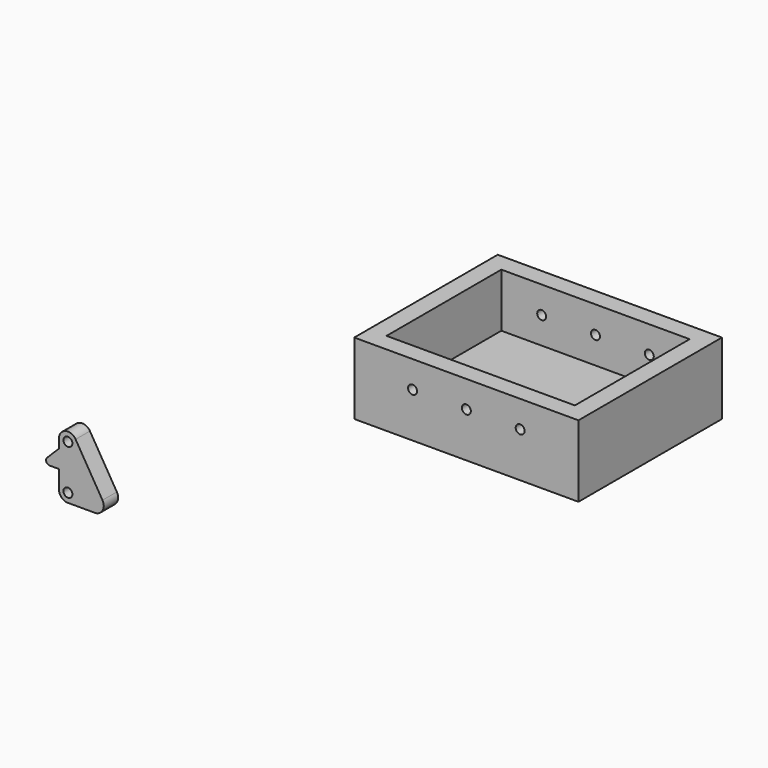
from build123d import *

# Parameters (mm, degrees)
F0_W      = 125
F0_H      = 100
F0_W_2    = 105
F0_H_2    = 80
F1_DEPTH  = 30
F2_R      = 2.5
F3_DEPTH  = 100.001
F4_W      = 125
F4_H      = 100
F4_W_2    = 105
F4_H_2    = 80
F5_DEPTH  = 10
F7_R      = 2.5
F8_DEPTH  = 10
F10_DEPTH = 10
F11_W     = 11.9066902784
F11_H     = 2
F11_W_2   = 5.1715728753
F11_W_3   = 11.2758645205
F12_DEPTH = 25


with BuildPart() as f1:
    # F0 (on Top) → F1 (new body)
    with BuildSketch(Plane.XY):
        with Locations((62.5, 50)):
            Rectangle(F0_W, F0_H)
        with Locations((62.5, 50)):
            Rectangle(F0_W_2, F0_H_2, mode=Mode.SUBTRACT)
    extrude(amount=F1_DEPTH)

    # F2 (on face) → F3 (cut, through all)
    with BuildSketch(Plane.XZ):
        with Locations((32.5, 15)):
            Circle(F2_R)
        with Locations((62.5, 15)):
            Circle(F2_R)
        with Locations((92.5, 15)):
            Circle(F2_R)
    extrude(amount=-F3_DEPTH, mode=Mode.SUBTRACT)

    # F4 (on face) → F5 (join)
    with BuildSketch(Plane(origin=(0, 0, 0), x_dir=(1, 0, 0), z_dir=(0, 0, -1))):
        with Locations((62.5, -50)):
            Rectangle(F4_W, F4_H)
        with Locations((62.5, -50)):
            Rectangle(F4_W_2, F4_H_2, mode=Mode.SUBTRACT)
        with Locations((62.5, -50)):
            Rectangle(F4_W_2, F4_H_2)
    extrude(amount=F5_DEPTH)


with BuildPart() as f8:
    # F7 (on Front) → F8 (new body)
    with BuildSketch(Plane.XZ):
        with BuildLine():
            ThreePointArc((-147.3962509632, -63.8523980975), (-153.0183835013, -61.6063022336), (-156.6837155918, -66.4248768747))
            Line((-156.6837155918, -66.4248768747), (-156.6837155918, -91.4248768747))
            ThreePointArc((-156.6837155918, -91.4248768747), (-155.2192494977, -94.9604107806), (-151.6837155918, -96.4248768747))
            Line((-151.6837155918, -96.4248768747), (-136.6837155918, -96.4248768747))
            ThreePointArc((-136.6837155918, -96.4248768747), (-132.332716058, -93.8883709496), (-132.3962509632, -88.8523980975))
            Line((-132.3962509632, -88.8523980975), (-147.3962509632, -63.8523980975))
        make_face()
        with Locations((-151.6837155918, -91.4248768747)):
            Circle(F7_R, mode=Mode.SUBTRACT)
        with Locations((-151.6837155918, -66.4248768747)):
            Circle(F7_R, mode=Mode.SUBTRACT)
    extrude(amount=F8_DEPTH)

    # F9 (on face) → F10 (join)
    with BuildSketch(Plane.XZ.offset(10)):
        with BuildLine():
            Line((-156.6837155918, -81.4248768747), (-156.6837155918, -71.4248768747))
            Line((-156.6837155918, -71.4248768747), (-163.2695020294, -78.0106633123))
            ThreePointArc((-163.2695020294, -78.0106633123), (-163.7030475321, -80.1902437394), (-161.855288467, -81.4248768747))
            Line((-161.855288467, -81.4248768747), (-156.6837155918, -81.4248768747))
        make_face()
    extrude(amount=-F10_DEPTH)

    # F11 (on face) → F12 (cut)
    with BuildSketch(Plane(origin=(0, 0, -81.4248768747), x_dir=(1, 0, 0), z_dir=(0, 0, -1))):
        with Locations((-167.8086336062, 7)):
            Rectangle(F11_W, F11_H)
        with Locations((-159.2695020294, 3)):
            Rectangle(F11_W_2, F11_H)
        with Locations((-159.2695020294, 7)):
            Rectangle(F11_W_2, F11_H)
        with Locations((-167.4932207273, 3)):
            Rectangle(F11_W_3, F11_H)
    extrude(amount=-F12_DEPTH, mode=Mode.SUBTRACT)


solid = Compound([f1.part, f8.part])
